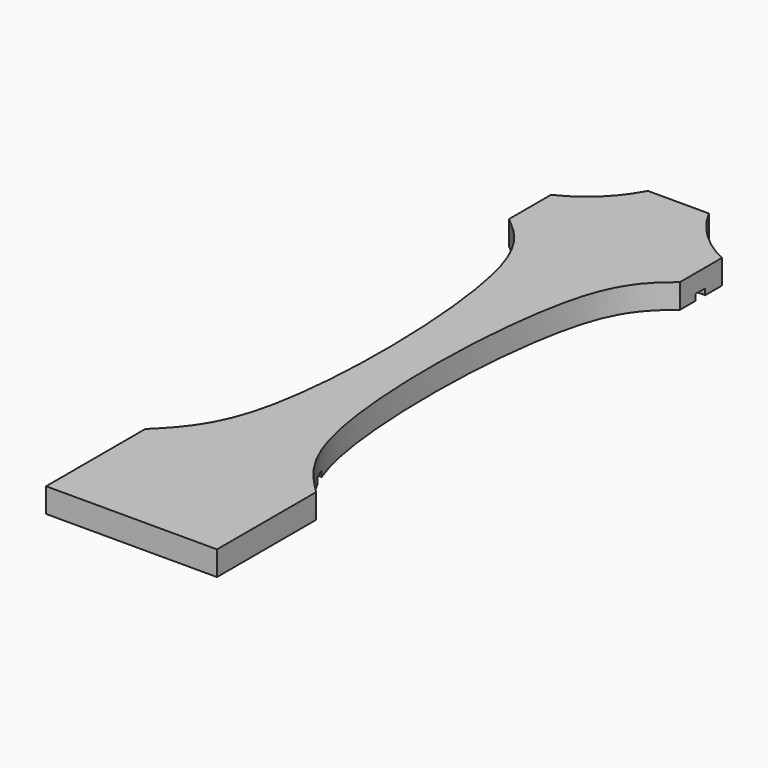
from build123d import *

# Parameters (mm, degrees)
F0_W     = 44.45
F0_H     = 31.75
F1_DEPTH = 177.8
F3_DEPTH = 44.451
F4_W     = 177.8
F4_H     = 25.4
F5_DEPTH = 66.04
F7_DEPTH = 25.4
F9_DEPTH = 25.4


# Not quite as in the source:
# - a pattern or mirror of a feature is missing from the dataset's text; its kind, count and spacing are read off the source's solid


with BuildPart() as f1:
    # F0 (on Front) → F1 (new body)
    with BuildSketch(Plane.XZ):
        Rectangle(F0_W, F0_H)
    extrude(amount=-F1_DEPTH)

    # F2 (on face) → F3 (cut, through all)
    with BuildSketch(Plane.YZ.offset(22.225)):
        with BuildLine():
            ThreePointArc((46.0375, -14.2875), (44.9149679849, -14.7524679849), (44.45, -15.875))
            Line((44.45, -15.875), (47.625, -15.875))
            ThreePointArc((47.625, -15.875), (47.1600320151, -14.7524679849), (46.0375, -14.2875))
        make_face()
        with BuildLine():
            ThreePointArc((46.0375, -14.2875), (47.1600320151, -14.7524679849), (47.625, -15.875))
            Line((47.625, -15.875), (47.625, -14.2875))
            Line((47.625, -14.2875), (46.0375, -14.2875))
        make_face()
        with BuildLine():
            Line((44.45, -14.2875), (44.45, -15.875))
            ThreePointArc((44.45, -15.875), (44.9149679849, -14.7524679849), (46.0375, -14.2875))
            Line((46.0375, -14.2875), (44.45, -14.2875))
        make_face()
        with BuildLine():
            ThreePointArc((157.1625, -14.2875), (156.0399679849, -14.7524679849), (155.575, -15.875))
            Line((155.575, -15.875), (158.75, -15.875))
            ThreePointArc((158.75, -15.875), (158.2850320151, -14.7524679849), (157.1625, -14.2875))
        make_face()
        with BuildLine():
            ThreePointArc((157.1625, -14.2875), (158.2850320151, -14.7524679849), (158.75, -15.875))
            Line((158.75, -15.875), (158.75, -14.2875))
            Line((158.75, -14.2875), (157.1625, -14.2875))
        make_face()
        with BuildLine():
            Line((155.575, -14.2875), (155.575, -15.875))
            ThreePointArc((155.575, -15.875), (156.0399679849, -14.7524679849), (157.1625, -14.2875))
            Line((157.1625, -14.2875), (155.575, -14.2875))
        make_face()
    extrude(amount=-F3_DEPTH, mode=Mode.SUBTRACT)

    # F4 (on face) → F5 (cut)
    with BuildSketch(Plane.YZ.offset(22.225)):
        with Locations((88.9, 3.175)):
            Rectangle(F4_W, F4_H)
    extrude(amount=-F5_DEPTH, mode=Mode.SUBTRACT)

    # F6 (on face) → F7 (cut)
    with BuildSketch(Plane.XY.offset(-9.525)):
        with BuildLine():
            add(Edge.make_bspline(
                [(-22.225, 150.5618393421), (-18.0890147105, 147.097734562), (-5.5252210375, 136.5748978803), (-3.6345620333, 50.7939916857), (-17.3552404375, 37.108562276), (-22.225, 32.2513133287)],
                knots=[0, 0, 0, 0, 0.2404536555, 0.7304209045, 1, 1, 1, 1], degree=3))
            Line((-22.225, 150.5618393421), (-22.225, 32.2513133287))
        make_face()
        with BuildLine():
            Line((22.225, 32.2513133287), (22.225, 150.5618393421))
            add(Edge.make_bspline(
                [(22.225, 150.5618393421), (18.0890147105, 147.097734562), (5.5252210375, 136.5748978803), (3.6345620333, 50.7939916857), (17.3552404375, 37.108562276), (22.225, 32.2513133287)],
                knots=[0, 0, 0, 0, 0.2404536555, 0.7304209045, 1, 1, 1, 1], degree=3))
        make_face()
    extrude(amount=-F7_DEPTH, mode=Mode.SUBTRACT)

    # F8 (on face) → F9 (cut)
    with BuildSketch(Plane.XY.offset(-9.525)):
        with BuildLine():
            Line((-22.225, 177.8), (-22.225, 164.1809196711))
            ThreePointArc((-22.225, 164.1809196711), (-13.9748413511, 169.8326284901), (-7.9310080037, 177.8))
            Line((-7.9310080037, 177.8), (-22.225, 177.8))
        make_face()
    f9 = extrude(amount=-F9_DEPTH, mode=Mode.SUBTRACT)

    # F9_copies: F9 across plane
    add(f9.mirror(Plane(origin=(0, 0, 0), x_dir=(0, 0, 1), z_dir=(1, 0, 0))), mode=Mode.SUBTRACT)


solid = f1.part
